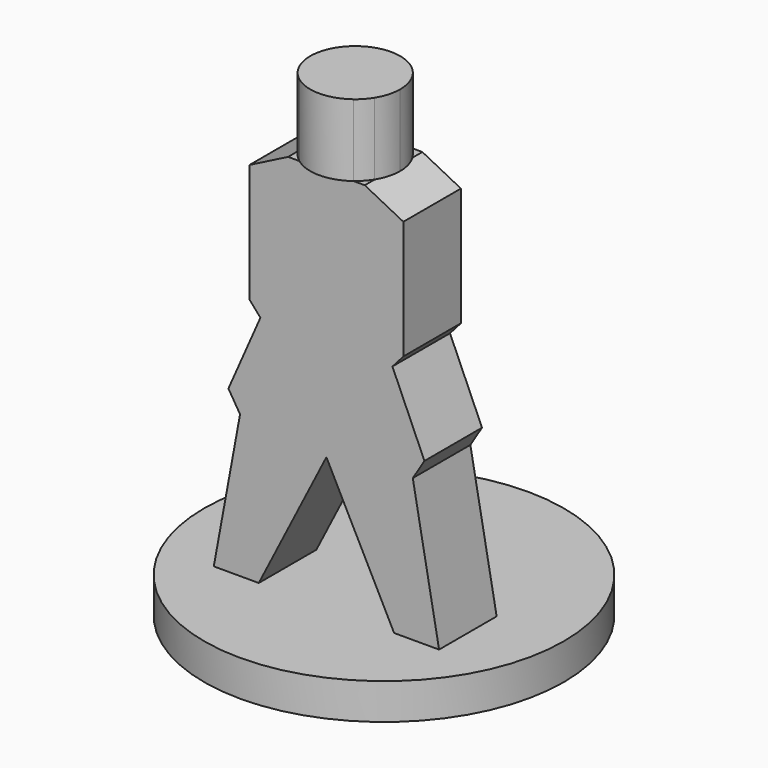
from build123d import *

# Parameters (mm, degrees)
F0_R     = 5
F1_DEPTH = 1
F3_DEPTH = 2
F5_DEPTH = 2


with BuildPart() as f1:
    # F0 (on Top) → F1 (new body)
    with BuildSketch(Plane.XY):
        Circle(F0_R)
    extrude(amount=F1_DEPTH)

    # F2 (on Front) → F3 (join)
    with BuildSketch(Plane.XZ):
        Polygon((-2.4001505226, 4.9579590559), (-3.1682769768, 0.7939044153), (-2.0160870627, 0.7332628593), (0, 4.6908766963), (0, 11.689173989), (-1.0660358239, 11.689173989), (-2.1373701748, 11.1433994025), (-2.1373701748, 7.848540321), (-1.8341623945, 7.5049051084), (-2.7235720772, 5.4835192859), align=None)
        Polygon((0, 11.689173989), (0, 4.6908766963), (2.0160870627, 0.7332628593), (3.1682769768, 0.7939044153), (2.4001505226, 4.9579590559), (2.7235720772, 5.4835192859), (1.8341623945, 7.5049051084), (2.1373701748, 7.848540321), (2.1373701748, 11.1433994025), (1.0660358239, 11.689173989), align=None)
    extrude(amount=F3_DEPTH)

    # F4 (on face) → F5 (join)
    with BuildSketch(Plane.XY.offset(11.689173989)):
        with BuildLine():
            Line((0.7512930037, 0), (0, 0))
            Line((0, 0), (0, -2))
            Line((0, -2), (0.7512930037, -2))
            ThreePointArc((0.7512930037, -2), (0.9249655721, -1.8419500388), (1.0660358239, -1.6542238146))
            Line((1.0660358239, -1.6542238146), (1.0660358239, -0.3457761854))
            ThreePointArc((1.0660358239, -0.3457761854), (0.9249655721, -0.1580499612), (0.7512930037, 0))
        make_face()
        with BuildLine():
            Line((-0.7512930037, 0), (0, 0))
            Line((0, 0), (0.7512930037, 0))
            ThreePointArc((0.7512930037, 0), (0, 0.25077623), (-0.7512930037, 0))
        make_face()
        with BuildLine():
            Line((0, -2), (0, 0))
            Line((0, 0), (-0.7512930037, 0))
            ThreePointArc((-0.7512930037, 0), (-0.9249655721, -0.1580499612), (-1.0660358239, -0.3457761854))
            Line((-1.0660358239, -0.3457761854), (-1.0660358239, -1.6542238146))
            ThreePointArc((-1.0660358239, -1.6542238146), (-0.9249655721, -1.8419500388), (-0.7512930037, -2))
            Line((-0.7512930037, -2), (0, -2))
        make_face()
        with BuildLine():
            Line((0.7512930037, -2), (0, -2))
            Line((0, -2), (-0.7512930037, -2))
            ThreePointArc((-0.7512930037, -2), (0, -2.25077623), (0.7512930037, -2))
        make_face()
        with BuildLine():
            ThreePointArc((1.25077623, -1), (1.2037054138, -0.6600964044), (1.0660358239, -0.3457761854))
            Line((1.0660358239, -0.3457761854), (1.0660358239, -1.6542238146))
            ThreePointArc((1.0660358239, -1.6542238146), (1.2037054138, -1.3399035956), (1.25077623, -1))
        make_face()
        with BuildLine():
            Line((-1.0660358239, -1.6542238146), (-1.0660358239, -0.3457761854))
            ThreePointArc((-1.0660358239, -0.3457761854), (-1.25077623, -1), (-1.0660358239, -1.6542238146))
        make_face()
    extrude(amount=F5_DEPTH)


solid = f1.part
